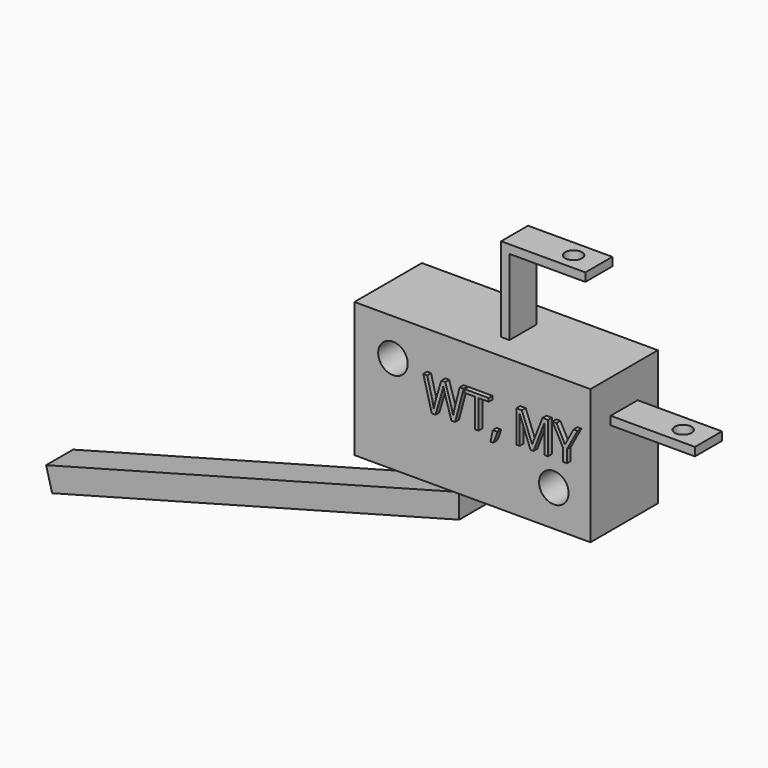
from build123d import *

# Parameters (mm, degrees)
F0_W          = 28
F0_H          = 16
F1_DEPTH      = 5
F2_R          = 1.7517571046
F3_DEPTH      = 10.001
F4_W          = 4
F4_H          = 1
F5_DEPTH      = 10
F6_W          = 1
F6_H          = 4
F7_DEPTH      = 10
F8_W          = 4
F8_H          = 1
F9_DEPTH      = 9
F10_R         = 1
F11_DEPTH     = 12.001
F12_R         = 1
F13_DEPTH     = 1
F14_W         = 0.9736078791
F14_H         = 4
F15_ANGLE     = 180
F14_W_2       = 0.722755678
F16_DEPTH     = 5
F17_T1_DEPTH  = 19.5803294212
F18_DEPTH     = 50
F19_TEXT_SIZE = 5.3328940541
F20_DEPTH     = 0.57123


# Not quite as in the source:
# - a fillet or chamfer that OpenCascade refuses, or shapes differently, is made with other operations: its cross-section is extruded or revolved along the edge and cut away or added
# - Text() gives the source's letters only with a copy of the font that has no kerning and outlines rounded to 1/6400 em; it was checked with that copy


with BuildPart() as f1:
    # F0 (on Front) → F1 (new body, symmetric)
    with BuildSketch(Plane.XZ):
        with Locations((14, -8)):
            Rectangle(F0_W, F0_H)
    extrude(amount=F1_DEPTH, both=True)

    # F2 (on face) → F3 (cut, through all)
    with BuildSketch(Plane.XZ.offset(5)):
        with Locations((4.5685651712, -4.4067171402)):
            Circle(F2_R)
        with Locations((23.6604232341, -11.7051443085)):
            Circle(F2_R)
    extrude(amount=-F3_DEPTH, mode=Mode.SUBTRACT)

    # F4 (on face) → F5 (join)
    with BuildSketch(Plane.YZ.offset(28)):
        with Locations((0, -4.5)):
            Rectangle(F4_W, F4_H)
    extrude(amount=F5_DEPTH)

    # F6 (on face) → F7 (join)
    with BuildSketch(Plane.XY):
        with Locations((15.5, 0)):
            Rectangle(F6_W, F6_H)
    extrude(amount=F7_DEPTH)

    # F8 (on face) → F9 (join)
    with BuildSketch(Plane.YZ.offset(16)):
        with Locations((0, 9.5)):
            Rectangle(F8_W, F8_H)
    extrude(amount=F9_DEPTH)

    # F10 (on face) → F11 (cut, through all)
    with BuildSketch(Plane.XY.offset(-4)):
        with Locations((35, 0)):
            Circle(F10_R)
    extrude(amount=-F11_DEPTH, mode=Mode.SUBTRACT)

    # F12 (on face) → F13 (cut, through all)
    with BuildSketch(Plane.XY.offset(10)):
        with Locations((22, 0)):
            Circle(F12_R)
    extrude(amount=-F13_DEPTH, mode=Mode.SUBTRACT)

    # F14 (on face) → F15 (revolve)
    with BuildSketch(Plane(origin=(0, 0, -16), x_dir=(1, 0, 0), z_dir=(0, 0, -1))):
        with Locations((7.3990991805, 0)):
            Rectangle(F14_W, F14_H)
    revolve(axis=Axis((6.9122952409, 0, -16), (0, 1, 0)), revolution_arc=F15_ANGLE)

    # F14 (on face) → F16 (join)
    with BuildSketch(Plane(origin=(0, 0, -16), x_dir=(1, 0, 0), z_dir=(0, 0, -1))):
        with Locations((9.6748749962, 0)):
            Rectangle(F14_W_2, F14_H)
    extrude(amount=F16_DEPTH)

    # F17: chamfer of 3 x 0.8038475773 on 1 edges, made by hand

    # F17_s2 → F17_t1 (cut)
    with BuildSketch(Plane.XZ.offset(-9.7901647106)):
        Polygon((9.3134971572, -18), (10.1173447345, -21), (9.3134971572, -21), align=None)
    extrude(amount=F17_T1_DEPTH, mode=Mode.SUBTRACT)

    # F18 (add): a face of the model
    f18_faces = [f1.faces().sort_by_distance(p)[0] for p in [
        (9.6748749962, 0, -19.3486804559),
    ]]
    extrude(f18_faces, amount=F18_DEPTH)

    # F19 (on face) → F20 (join)
    with BuildSketch(Plane.XZ.offset(5)):
        with Locations((8.5531910881, -8.2781147212)):
            Text('WT, MY', F19_TEXT_SIZE, font='Open Sans', text_align=(TextAlign.LEFT, TextAlign.BOTTOM))
    extrude(amount=F20_DEPTH)


solid = f1.part
